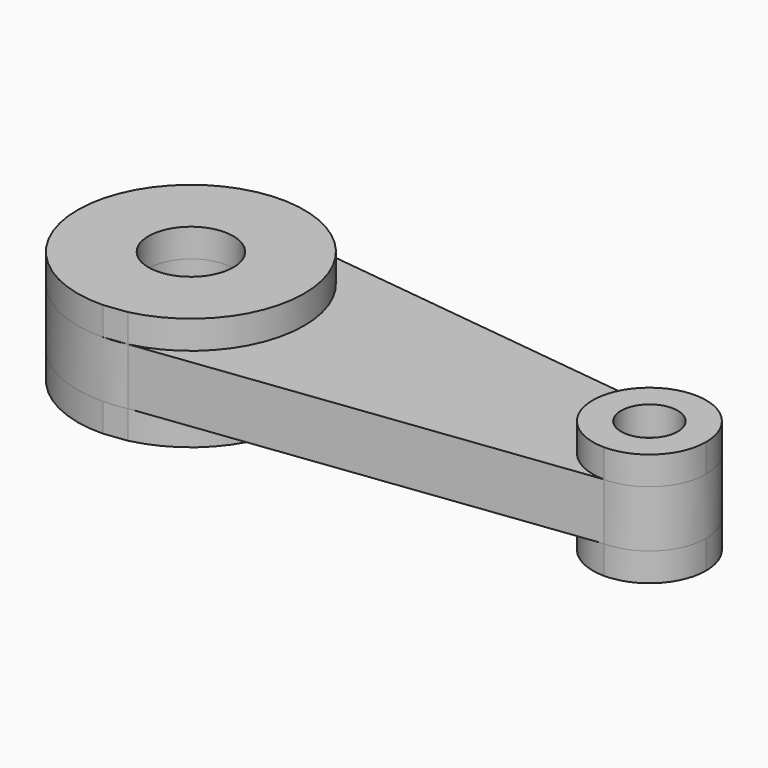
from build123d import *

# Parameters (mm, degrees)
F0_R          = 9.5051197762
F1_DEPTH      = 12.7
F1_DEPTH_BACK = 12.7
F0_R_2        = 6.35
F2_DEPTH      = 6.35
F2_DEPTH_BACK = 6.35
F3_R          = 12.7
F4_DEPTH      = 12.7


with BuildPart() as f1:
    # F0 (on Top) → F1 (new body, two sides)
    with BuildSketch(Plane.XY) as f1_sk:
        with BuildLine():
            ThreePointArc((-63.0856611977, -24.7605061219), (-48.8871011462, -15.8319673643), (-43.3493469753, 0))
            ThreePointArc((-43.3493469753, 0), (-48.3861185924, 15.1821912064), (-61.498869009, 24.3431832196))
            ThreePointArc((-61.498869009, 24.3431832196), (-93.9227433709, 3.3852789998), (-68.187418541, -25.393783421))
            Line((-68.187418541, -25.393783421), (-63.0856611977, -24.7605061219))
        make_face()
        with Locations((-68.7493469753, 0)):
            Circle(F0_R, mode=Mode.SUBTRACT)
    extrude(amount=F1_DEPTH)
    extrude(f1_sk.sketch, amount=-F1_DEPTH_BACK)

    # F3 (on face) → F4 (cut)
    with BuildSketch(Plane(origin=(0, 0, -12.7), x_dir=(1, 0, 0), z_dir=(0, 0, -1))):
        with Locations((-68.7493469753, 0)):
            Circle(F3_R)
    extrude(amount=-F4_DEPTH, mode=Mode.SUBTRACT)


with BuildPart() as f1b:
    # F0 (on Top) → F1, piece 2 (new body, two sides)
    with BuildSketch(Plane.XY) as f1_2_sk:
        with BuildLine():
            Line((36.2084881778, 12.5195501056), (34.9897814236, 12.6670266309))
            ThreePointArc((34.9897814236, 12.6670266309), (21.383458511, 0.4575815704), (34.0752124917, -12.7))
            ThreePointArc((34.0752124917, -12.7), (43.0554686128, -8.9802561211), (46.7752124917, 0))
            ThreePointArc((46.7752124917, 0), (43.7804327678, 8.1913795782), (36.2084881778, 12.5195501056))
        make_face()
        with Locations((34.0752124917, 0)):
            Circle(F0_R_2, mode=Mode.SUBTRACT)
    extrude(amount=F1_DEPTH)
    extrude(f1_2_sk.sketch, amount=-F1_DEPTH_BACK)


with BuildPart() as f2:
    # F0 (on Top) → F2 (new body, two sides)
    with BuildSketch(Plane.XY) as f2_sk:
        with BuildLine():
            ThreePointArc((-63.0856611977, -24.7605061219), (-48.8871011462, -15.8319673643), (-43.3493469753, 0))
            ThreePointArc((-43.3493469753, 0), (-48.3861185924, 15.1821912064), (-61.498869009, 24.3431832196))
            ThreePointArc((-61.498869009, 24.3431832196), (-93.9227433709, 3.3852789998), (-68.187418541, -25.393783421))
            Line((-68.187418541, -25.393783421), (-63.0856611977, -24.7605061219))
        make_face()
        with Locations((-68.7493469753, 0)):
            Circle(F0_R, mode=Mode.SUBTRACT)
        with BuildLine():
            ThreePointArc((-61.498869009, 24.3431832196), (-48.3861185924, 15.1821912064), (-43.3493469753, 0))
            ThreePointArc((-43.3493469753, 0), (-48.8871011462, -15.8319673643), (-63.0856611977, -24.7605061219))
            Line((-63.0856611977, -24.7605061219), (34.0752124917, -12.7))
            ThreePointArc((34.0752124917, -12.7), (21.383458511, 0.4575815704), (34.9897814236, 12.6670266309))
            Line((34.9897814236, 12.6670266309), (-61.498869009, 24.3431832196))
        make_face()
        with BuildLine():
            ThreePointArc((-68.187418541, -25.393783421), (-65.6204768736, -25.2065501782), (-63.0856611977, -24.7605061219))
            Line((-63.0856611977, -24.7605061219), (-68.187418541, -25.393783421))
        make_face()
        with BuildLine():
            Line((36.2084881778, 12.5195501056), (34.9897814236, 12.6670266309))
            ThreePointArc((34.9897814236, 12.6670266309), (21.383458511, 0.4575815704), (34.0752124917, -12.7))
            ThreePointArc((34.0752124917, -12.7), (43.0554686128, -8.9802561211), (46.7752124917, 0))
            ThreePointArc((46.7752124917, 0), (43.7804327678, 8.1913795782), (36.2084881778, 12.5195501056))
        make_face()
        with Locations((34.0752124917, 0)):
            Circle(F0_R_2, mode=Mode.SUBTRACT)
        with BuildLine():
            ThreePointArc((36.2084881778, 12.5195501056), (35.60091775, 12.6080221869), (34.9897814236, 12.6670266309))
            Line((34.9897814236, 12.6670266309), (36.2084881778, 12.5195501056))
        make_face()
    extrude(amount=F2_DEPTH)
    extrude(f2_sk.sketch, amount=-F2_DEPTH_BACK)


solid = Compound([f1.part, f1b.part, f2.part])
